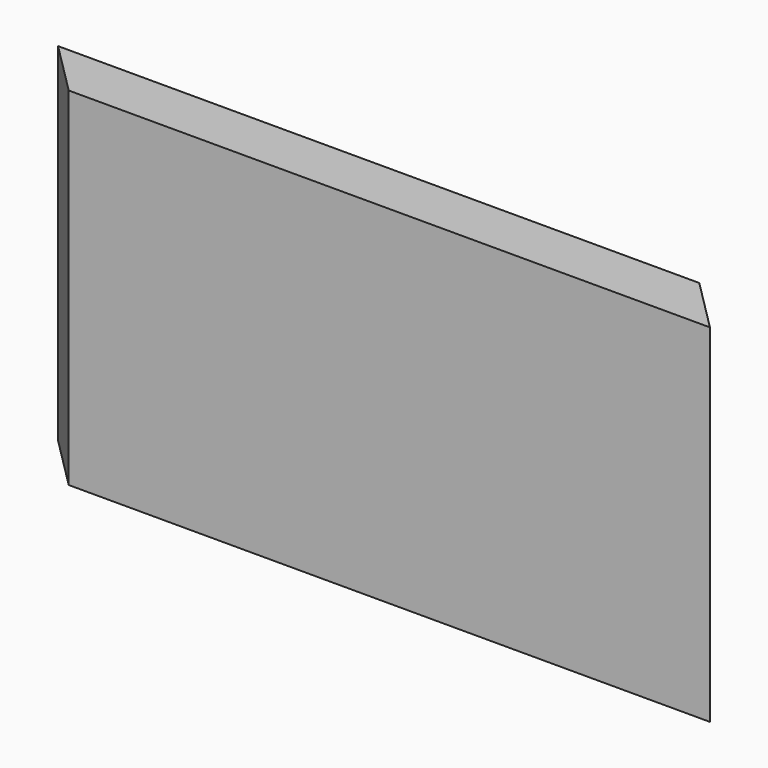
from build123d import *

# Parameters (mm, degrees)
F0_W     = 165.1
F0_H     = 82.55
F1_DEPTH = 12.7
F2_SIZE  = 12.69999


# Not quite as in the source:
# - a fillet or chamfer is up to 0.001 mm smaller than in the source, because OpenCascade refuses the exact size


with BuildPart() as f1:
    # F0 (on Front) → F1 (new body)
    with BuildSketch(Plane.XZ):
        with Locations((-17.9753675056, -2.1604858339)):
            Rectangle(F0_W, F0_H)
    extrude(amount=F1_DEPTH)

    # F2 (size 12.7 in the source; OpenCascade refuses exactly that, so slightly less here)
    f2_edges = [f1.edges().sort_by_distance(p)[0] for p in [
        (64.574632, 0, -2.160486),
        (-100.525368, -12.7, -2.160486),
    ]]
    chamfer(f2_edges, length=F2_SIZE)


solid = f1.part
